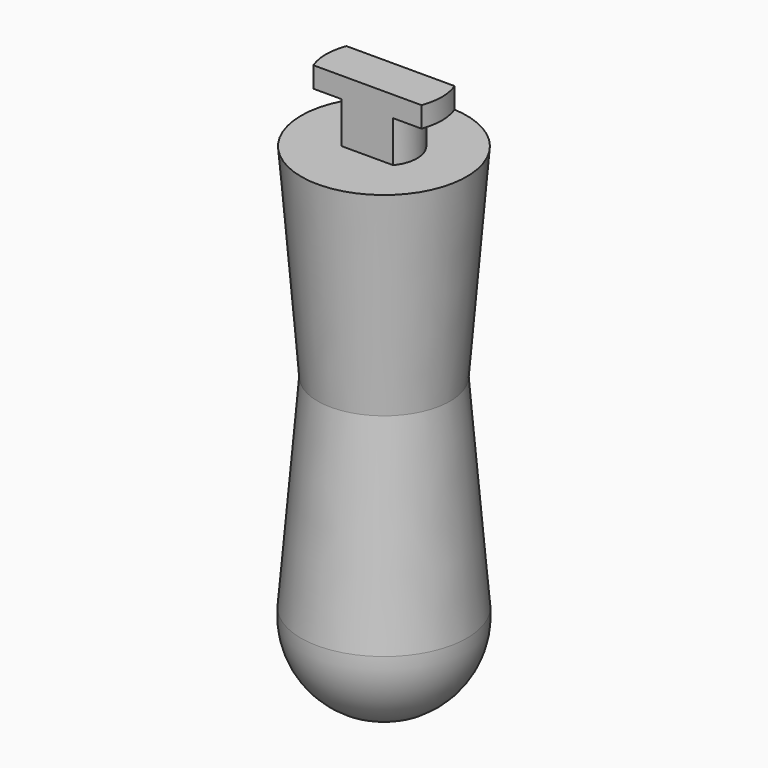
from build123d import *

# Parameters (mm, degrees)
F3_DEPTH = 9.525


with BuildPart() as f1:
    # F0 (on Front) → F1 (revolve)
    with BuildSketch(Plane.XZ):
        Polygon((0, -31.1628540011), (0, 0), (-5.08, 0), (-12.7, 0), (-10.16, -31.1628540011), align=None)
        Polygon((-5.08, 0), (0, 0), (0, 9.525), (-8.89, 9.525), (-8.89, 6.35), (-5.08, 6.35), align=None)
        Polygon((0, -62.3257080022), (0, -31.1628540011), (-10.16, -31.1628540011), (-12.7635, -62.3257080022), align=None)
        with BuildLine():
            Line((0, -76.2), (0, -62.3257080022))
            Line((0, -62.3257080022), (-12.7635, -62.3257080022))
            ThreePointArc((-12.7635, -62.3257080022), (-9.4260663944, -72.0634388747), (0, -76.2))
        make_face()
    revolve(axis=Axis((0, 0, -38.1), (0, 0, -1)))

    # F2 (on face) → F3 (cut, through all)
    with BuildSketch(Plane.XY.offset(9.525)):
        with BuildLine():
            ThreePointArc((8.3037024874, 3.175), (0, 8.89), (-8.3037024874, 3.175))
            Line((-8.3037024874, 3.175), (8.3037024874, 3.175))
        make_face()
        with BuildLine():
            Line((8.3037024874, -3.175), (-8.3037024874, -3.175))
            ThreePointArc((-8.3037024874, -3.175), (0, -8.89), (8.3037024874, -3.175))
        make_face()
        with BuildLine():
            ThreePointArc((10.9695693512, 3.175), (0, 11.4198107144), (-10.9695693512, 3.175))
            Line((-10.9695693512, 3.175), (-8.3037024874, 3.175))
            ThreePointArc((-8.3037024874, 3.175), (0, 8.89), (8.3037024874, 3.175))
            Line((8.3037024874, 3.175), (10.9695693512, 3.175))
        make_face()
        with BuildLine():
            Line((-8.3037024874, -3.175), (-10.9695693512, -3.175))
            ThreePointArc((-10.9695693512, -3.175), (0, -11.4198107144), (10.9695693512, -3.175))
            Line((10.9695693512, -3.175), (8.3037024874, -3.175))
            ThreePointArc((8.3037024874, -3.175), (0, -8.89), (-8.3037024874, -3.175))
        make_face()
        with BuildLine():
            Line((-8.3037024874, 3.175), (-10.9695693512, 3.175))
            ThreePointArc((-10.9695693512, 3.175), (-11.4198107144, 0), (-10.9695693512, -3.175))
            Line((-10.9695693512, -3.175), (-8.3037024874, -3.175))
            ThreePointArc((-8.3037024874, -3.175), (-8.89, 0), (-8.3037024874, 3.175))
        make_face()
        with BuildLine():
            ThreePointArc((11.4198107144, 0), (11.3066901072, 1.6033825405), (10.9695693512, 3.175))
            Line((10.9695693512, 3.175), (8.3037024874, 3.175))
            ThreePointArc((8.3037024874, 3.175), (8.7421969525, 1.6143396307), (8.89, 0))
            ThreePointArc((8.89, 0), (8.7421969525, -1.6143396307), (8.3037024874, -3.175))
            Line((8.3037024874, -3.175), (10.9695693512, -3.175))
            ThreePointArc((10.9695693512, -3.175), (11.3066901072, -1.6033825405), (11.4198107144, 0))
        make_face()
    extrude(amount=-F3_DEPTH, mode=Mode.SUBTRACT)


solid = f1.part
